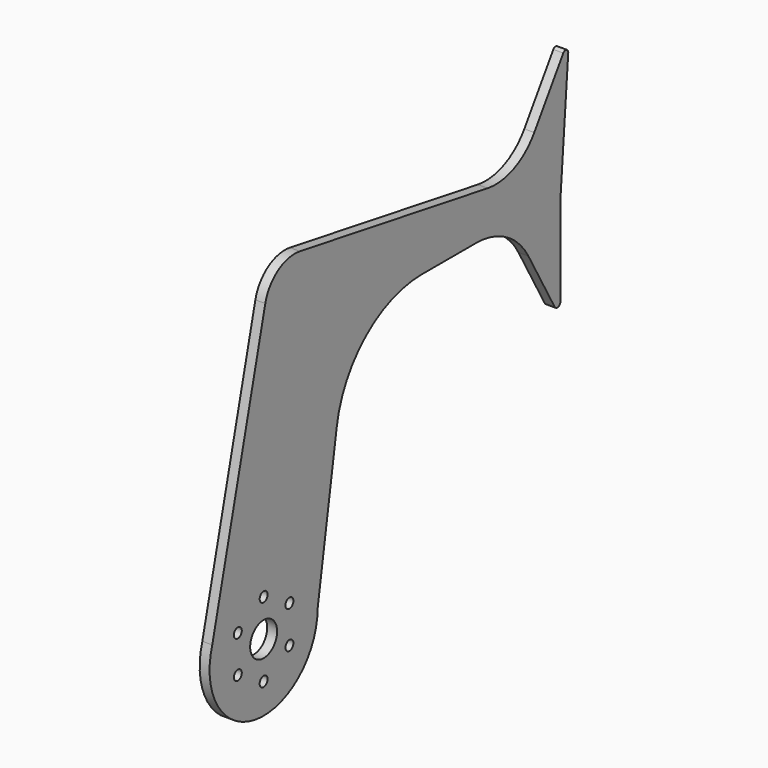
from build123d import *

# Parameters (mm, degrees)
F1_DEPTH = 6.35
F2_DEPTH = 6.35
F0_R     = 10.7670897693
F5_DEPTH = 6.35
F6_D     = 6.35


# Not quite as in the source:
# - a feature of the source that left no trace in its solid (it failed there, or was rolled back) is left out


with BuildPart() as f1:
    # F0 (on Right) → F1 (new body)
    with BuildSketch(Plane.YZ):
        with BuildLine():
            ThreePointArc((-1.5825573364, -153.9491721496), (-1.5826429755, -154.035180638), (-1.5828998925, -154.1211887854))
            Line((-1.5828998925, -154.1211887854), (13.683948877, -58.1386835494))
            ThreePointArc((13.683948877, -58.1386835494), (37.0236297514, -16.510860014), (81.800944289, 0))
            Line((81.800944289, 0), (125.0803981306, 0))
            ThreePointArc((125.0803981306, 0), (149.2715136598, -6.5386249673), (166.8746197449, -24.3738245223))
            Line((166.8746197449, -24.3738245223), (187.8910975974, -61.5208026845))
            ThreePointArc((187.8910975974, -61.5208026845), (190.6720383022, -62.6941019502), (192.5146989034, -60.3035237191))
            Line((192.5146989034, -60.3035237191), (192.5146989034, -2.1215420715))
            Line((192.5146989034, -2.1215420715), (198.7226175975, 77.2382490494))
            ThreePointArc((198.7226175975, 77.2382490494), (197.2700771229, 79.4482102797), (194.7679715475, 78.5918983278))
            Line((194.7679715475, 78.5918983278), (171.5573410493, 43.2821044094))
            ThreePointArc((171.5573410493, 43.2821044094), (155.3522029023, 29.6366600871), (134.3221352203, 27.0791405068))
            Line((134.3221352203, 27.0791405068), (-15.8528228172, 52.6105930486))
            ThreePointArc((-15.8528228172, 52.6105930486), (-33.2247403603, 48.9627075804), (-43.4379661828, 34.4444223576))
            Line((-43.4379661828, 34.4444223576), (-85.8287484087, -140.5429926023))
            ThreePointArc((-85.8287484087, -140.5429926023), (-37.9848929099, -111.2960762471), (-1.5825573364, -153.9491721496))
        make_face()
    extrude(amount=F1_DEPTH)

    # F0 (on Right) → F2 (join)
    with BuildSketch(Plane.YZ):
        with BuildLine():
            ThreePointArc((-1.5825573364, -153.9491721496), (-1.5826429755, -154.035180638), (-1.5828998925, -154.1211887854))
            Line((-1.5828998925, -154.1211887854), (13.683948877, -58.1386835494))
            ThreePointArc((13.683948877, -58.1386835494), (37.0236297514, -16.510860014), (81.800944289, 0))
            Line((81.800944289, 0), (125.0803981306, 0))
            ThreePointArc((125.0803981306, 0), (149.2715136598, -6.5386249673), (166.8746197449, -24.3738245223))
            Line((166.8746197449, -24.3738245223), (187.8910975974, -61.5208026845))
            ThreePointArc((187.8910975974, -61.5208026845), (190.6720383022, -62.6941019502), (192.5146989034, -60.3035237191))
            Line((192.5146989034, -60.3035237191), (192.5146989034, -2.1215420715))
            Line((192.5146989034, -2.1215420715), (198.7226175975, 77.2382490494))
            ThreePointArc((198.7226175975, 77.2382490494), (197.2700771229, 79.4482102797), (194.7679715475, 78.5918983278))
            Line((194.7679715475, 78.5918983278), (171.5573410493, 43.2821044094))
            ThreePointArc((171.5573410493, 43.2821044094), (155.3522029023, 29.6366600871), (134.3221352203, 27.0791405068))
            Line((134.3221352203, 27.0791405068), (-15.8528228172, 52.6105930486))
            ThreePointArc((-15.8528228172, 52.6105930486), (-33.2247403603, 48.9627075804), (-43.4379661828, 34.4444223576))
            Line((-43.4379661828, 34.4444223576), (-85.8287484087, -140.5429926023))
            ThreePointArc((-85.8287484087, -140.5429926023), (-37.9848929099, -111.2960762471), (-1.5825573364, -153.9491721496))
        make_face()
    extrude(amount=F2_DEPTH)

    # F0 (on Right) → F5 (join)
    with BuildSketch(Plane.YZ):
        with BuildLine():
            ThreePointArc((-85.8287484087, -140.5429926023), (-51.6446777228, -196.588666929), (-1.5828998925, -154.1211887854))
            ThreePointArc((-1.5828998925, -154.1211887854), (-1.5826429755, -154.035180638), (-1.5825573364, -153.9491721496))
            ThreePointArc((-1.5825573364, -153.9491721496), (-37.9848929099, -111.2960762471), (-85.8287484087, -140.5429926023))
        make_face()
        with Locations((-44.772322165, -153.9491721496)):
            Circle(F0_R, mode=Mode.SUBTRACT)
    extrude(amount=F5_DEPTH)

    # F6 (through all)
    with Locations(Plane(origin=(0, 0, 0), x_dir=(0, 1, 0), z_dir=(-1, 0, 0))):
        with Locations((-44.772322165, 130.1366721496), (-24.1500922374, 142.0429221496), (-24.1500922374, 165.8554221496), (-44.772322165, 177.7616721496), (-65.3945520927, 165.8554221496), (-65.3945520927, 142.0429221496)):
            Hole(F6_D / 2)


solid = f1.part
